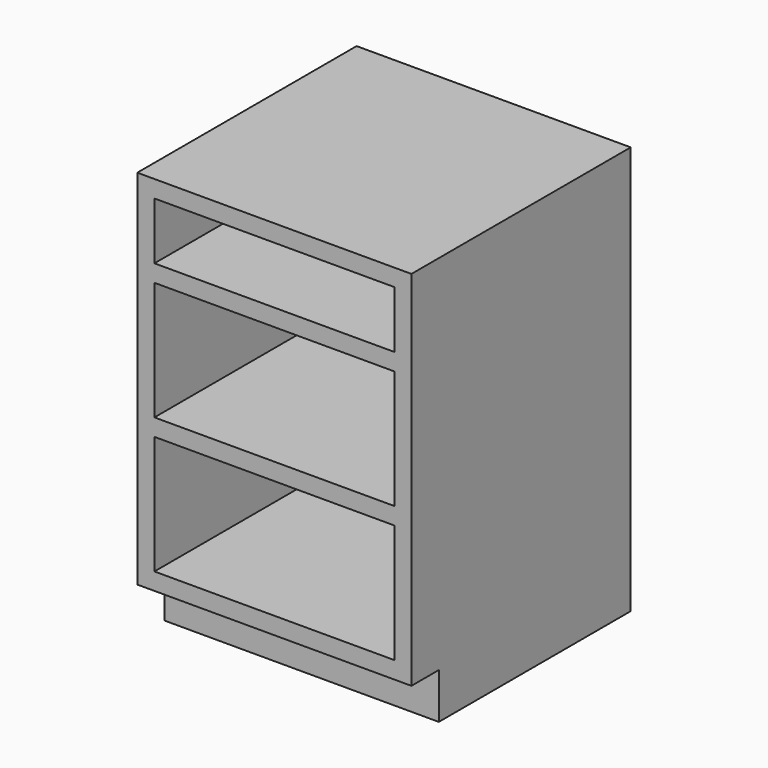
from build123d import *

# Parameters (mm, degrees)
F1_DEPTH = 609.6
F2_W     = 533.4
F2_H     = 127
F2_H_2   = 263.525
F3_DEPTH = 596.9


# Not quite as in the source:
# - a feature names something its author has since deleted; it is built from what else it names


with BuildPart() as f1:
    # F0 (on Right) → F1 (new body)
    with BuildSketch(Plane.YZ):
        Polygon((-533.4, 0), (0, 0), (0, 908.05), (-609.6, 908.05), (-609.6, 101.6), (-533.4, 101.6), align=None)
    extrude(amount=F1_DEPTH)

    # F2 (on face) → F3 (cut)
    with BuildSketch(Plane.XZ.offset(609.6)):
        with Locations((304.8, 806.45)):
            Rectangle(F2_W, F2_H)
        with Locations((304.8, 573.0875)):
            Rectangle(F2_W, F2_H_2)
        with Locations((304.8, 271.4625)):
            Rectangle(F2_W, F2_H_2)
    extrude(amount=-F3_DEPTH, mode=Mode.SUBTRACT)


solid = f1.part
